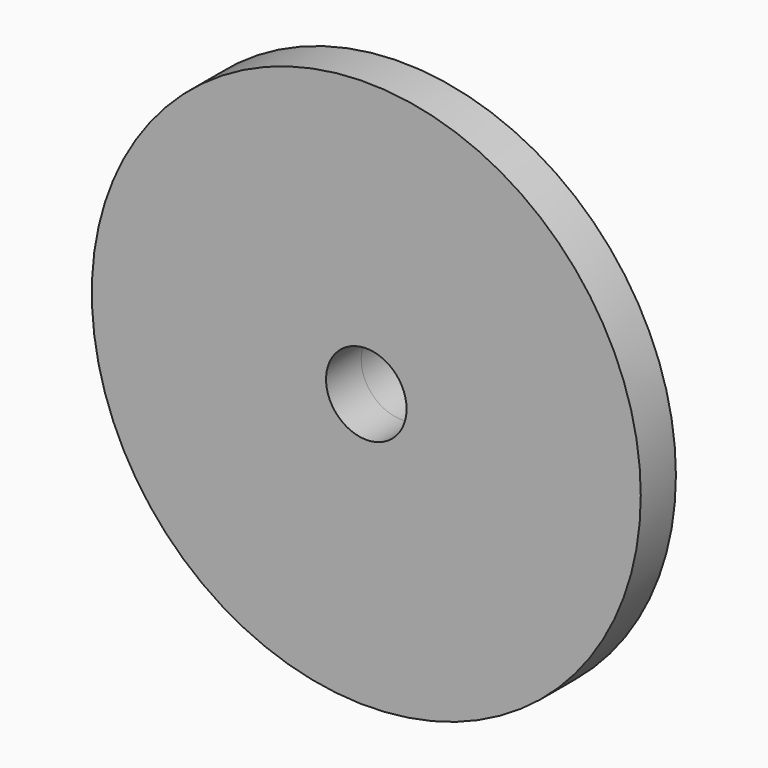
from build123d import *
from build123d import SkipClean  # not in build123d's __all__

# Parameters (mm, degrees)
F0_R     = 15
F1_DEPTH = 2.4
F2_R     = 2.2
F3_DEPTH = 2.401
F4_R     = 3
F4_R_2   = 2.2
F5_DEPTH = 5


with BuildPart() as f1:
    # F0 (on Front) → F1 (new body)
    with BuildSketch(Plane.XZ):
        Circle(F0_R)
    extrude(amount=F1_DEPTH)

    # F2 (on face) → F3 (cut, through all)
    with BuildSketch(Plane.XZ.offset(2.4)):
        Circle(F2_R)
    extrude(amount=-F3_DEPTH, mode=Mode.SUBTRACT)

    # F4 (on face) → F5 (join)
    with BuildSketch(Plane(origin=(0, 0, 0), x_dir=(-1, 0, 0), z_dir=(0, 1, 0))):
        Circle(F4_R)
        Circle(F4_R_2, mode=Mode.SUBTRACT)
        with BuildLine():
            ThreePointArc((-2, 7.2284161474), (-5.3033008589, 5.3033008589), (-7.2284161474, 2))
            Line((-7.2284161474, 2), (-6.1846584384, 2))
            ThreePointArc((-6.1846584384, 2), (-4.5961940777, 4.5961940777), (-2, 6.1846584384))
            Line((-2, 6.1846584384), (-2, 7.2284161474))
        make_face()
        with BuildLine():
            Line((-2, -7.2284161474), (-2, -6.1846584384))
            ThreePointArc((-2, -6.1846584384), (-4.5961940777, -4.5961940777), (-6.1846584384, -2))
            Line((-6.1846584384, -2), (-7.2284161474, -2))
            ThreePointArc((-7.2284161474, -2), (-5.3033008589, -5.3033008589), (-2, -7.2284161474))
        make_face()
        with BuildLine():
            Line((2, 7.2284161474), (2, 6.1846584384))
            ThreePointArc((2, 6.1846584384), (4.5961940777, 4.5961940777), (6.1846584384, 2))
            Line((6.1846584384, 2), (7.2284161474, 2))
            ThreePointArc((7.2284161474, 2), (5.3033008589, 5.3033008589), (2, 7.2284161474))
        make_face()
        with BuildLine():
            ThreePointArc((6.1846584384, -2), (4.5961940777, -4.5961940777), (2, -6.1846584384))
            Line((2, -6.1846584384), (2, -7.2284161474))
            ThreePointArc((2, -7.2284161474), (5.3033008589, -5.3033008589), (7.2284161474, -2))
            Line((7.2284161474, -2), (6.1846584384, -2))
        make_face()
    with SkipClean():  # cleaning this boolean's faces spoils the solid; the shape is the same uncleaned
        extrude(amount=F5_DEPTH)


solid = f1.part
